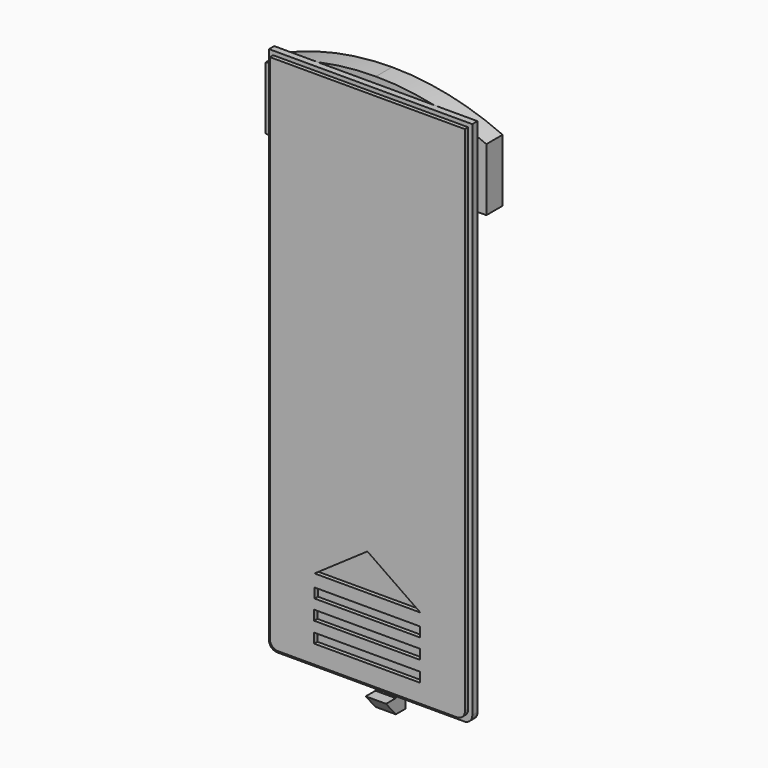
from build123d import *

# Parameters (mm, degrees)
F0_W      = 25
F0_H      = 65
F1_DEPTH  = 0.8
F2_W      = 24
F2_H      = 64
F3_DEPTH  = 0.5
F4_R      = 1
F4_2_R    = 1
F5_W      = 6.5
F5_H      = 1.2
F6_DEPTH  = 0.7
F8_DEPTH  = 1.25
F9_W      = 2.5
F9_H      = 1.5
F10_DEPTH = 3.5
F12_DEPTH = 1.25
F14_DEPTH = 2.5


with BuildPart() as f1:
    # F0 (on Front) → F1 (new body)
    with BuildSketch(Plane.XZ):
        Rectangle(F0_W, F0_H)
    extrude(amount=F1_DEPTH)

    # F4
    f4_edges = [f1.edges().sort_by_distance(p)[0] for p in [
        (12.5, -0.4, -32.5),
        (-12.5, -0.4, -32.5),
    ]]
    fillet(f4_edges, radius=F4_R)

    # F7 (on Right) → F8 (join, symmetric)
    with BuildSketch(Plane.YZ):
        Polygon((0, -30.5), (0, -32.5), (3, -32.5), align=None)
    extrude(amount=F8_DEPTH, both=True)

    # F9 (on face) → F10 (join)
    with BuildSketch(Plane(origin=(0, 0, -32.5), x_dir=(1, 0, 0), z_dir=(0, 0, -1))):
        with Locations((0, -2.25)):
            Rectangle(F9_W, F9_H)
    extrude(amount=F10_DEPTH)

    # F11 (on Right) → F12 (join, symmetric)
    with BuildSketch(Plane.YZ):
        Polygon((1.5, -36), (1.5, -34.25), (0, -34.25), align=None)
    extrude(amount=F12_DEPTH, both=True)


with BuildPart() as f3:
    # F2 (on face) → F3 (new body)
    with BuildSketch(Plane.XZ.offset(0.8)):
        Rectangle(F2_W, F2_H)
    extrude(amount=F3_DEPTH)

    # F4#2
    f4_2_edges = [f3.edges().sort_by_distance(p)[0] for p in [
        (12, -1.05, -32),
        (-12, -1.05, -32),
    ]]
    fillet(f4_2_edges, radius=F4_2_R)

    # F5 (on face) → F6 (cut)
    with BuildSketch(Plane.XZ.offset(1.3)):
        Polygon((-6.5, -22.1242941916), (0, -22.1242941916), (6.5, -22.1242941916), (0, -17.6242941916), align=None)
        with Locations((-3.2513196841, -24.2404304445)):
            Rectangle(F5_W, F5_H)
        with Locations((3.2486803159, -24.2404304445)):
            Rectangle(F5_W, F5_H)
        with Locations((3.1881782691, -26.6605243087)):
            Rectangle(F5_W, F5_H)
        with Locations((-3.3118217309, -26.6605243087)):
            Rectangle(F5_W, F5_H)
        with Locations((-3.3118230551, -29.1411206126)):
            Rectangle(F5_W, F5_H)
        with Locations((3.1881769449, -29.1411206126)):
            Rectangle(F5_W, F5_H)
    extrude(amount=-F6_DEPTH, mode=Mode.SUBTRACT)


with BuildPart() as f14:
    # F13 (on Front) → F14 (new body)
    with BuildSketch(Plane.XZ):
        with BuildLine():
            ThreePointArc((-11.557778761, 30.3686572288), (-5.8757523748, 31.957990015), (0, 32.4936546385))
            ThreePointArc((0, 32.4936546385), (5.8757523748, 31.957990015), (11.557778761, 30.3686572288))
            Line((11.557778761, 30.3686572288), (11.557778761, 22.671321407))
            Line((11.557778761, 22.671321407), (13.5913705453, 22.671321407))
            Line((13.5913705453, 22.671321407), (13.5913705453, 30.3686572288))
            ThreePointArc((13.5913705453, 30.3686572288), (6.9489351887, 32.5375628301), (0, 33.2713194085))
            ThreePointArc((0, 33.2713194085), (-6.9489351887, 32.5375628301), (-13.5913705453, 30.3686572288))
            Line((-13.5913705453, 30.3686572288), (-13.5913705453, 22.671321407))
            Line((-13.5913705453, 22.671321407), (-11.557778761, 22.671321407))
            Line((-11.557778761, 22.671321407), (-11.557778761, 30.3686572288))
        make_face()
    extrude(amount=-F14_DEPTH)


solid = Compound([f1.part, f3.part, f14.part])
